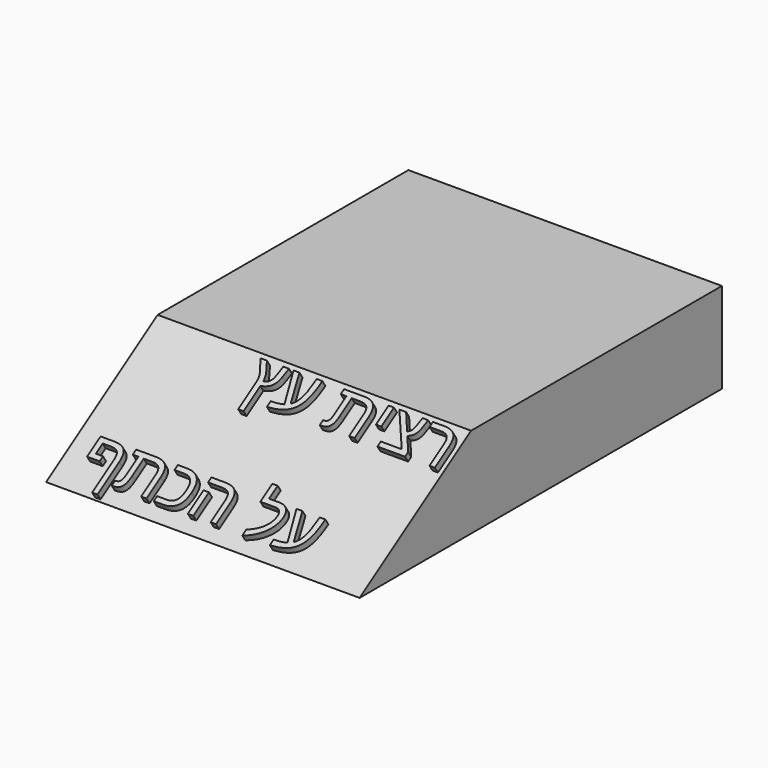
from build123d import *

# Parameters (mm, degrees)
F1_DEPTH     = 571.5
F2_TEXT_SIZE = 218.7222222222
F3_DEPTH     = 25.4
F4_TEXT_SIZE = 123.4722222222
F5_DEPTH     = 25.4


# Not quite as in the source:
# - Text() gives the source's letters only with a copy of the font that has no kerning and outlines rounded to 1/6400 em; it was checked with that copy


with BuildPart() as f1:
    # F0 (on Right) → F1 (new body, symmetric)
    with BuildSketch(Plane.YZ):
        Polygon((342.1609172821, -998.8214373589), (342.1609172821, -668.6214373589), (-800.8390827179, -668.6214373589), (-1308.8390827179, -998.8214373589), align=None)
    extrude(amount=F1_DEPTH, both=True)

    # F2 (on face) → F3 (join)
    with BuildSketch(Plane(origin=(0, 67.6621594622, -104.0956299418), x_dir=(1, 0, 0), z_dir=(0, -0.5449883506, 0.8384436163))):
        with Locations((-168.4304427083, -1193.3293109078)):
            Text('ץע תיצר', F2_TEXT_SIZE, font='Arimo', text_align=(TextAlign.LEFT, TextAlign.BOTTOM))
        with Locations((-497.083357593, -1592.4172928641)):
            Text('ףתכה לע', F2_TEXT_SIZE, font='Arimo', text_align=(TextAlign.LEFT, TextAlign.BOTTOM))
    extrude(amount=F3_DEPTH)

    # F4 (on face) → F5 (cut)
    with BuildSketch(Plane(origin=(0, 342.1609172821, 0), x_dir=(-1, 0, 0), z_dir=(0, 1, 0))):
        with Locations((-380.8511233099, -951.0169020633)):
            Text('דרעמ', F4_TEXT_SIZE, font='Arimo', text_align=(TextAlign.LEFT, TextAlign.BOTTOM))
        with Locations((44.3904089841, -897.6128534518)):
            Text("16 'גוא", F4_TEXT_SIZE, font='Arimo', text_align=(TextAlign.LEFT, TextAlign.BOTTOM))
    extrude(amount=-F5_DEPTH, mode=Mode.SUBTRACT)


solid = f1.part
